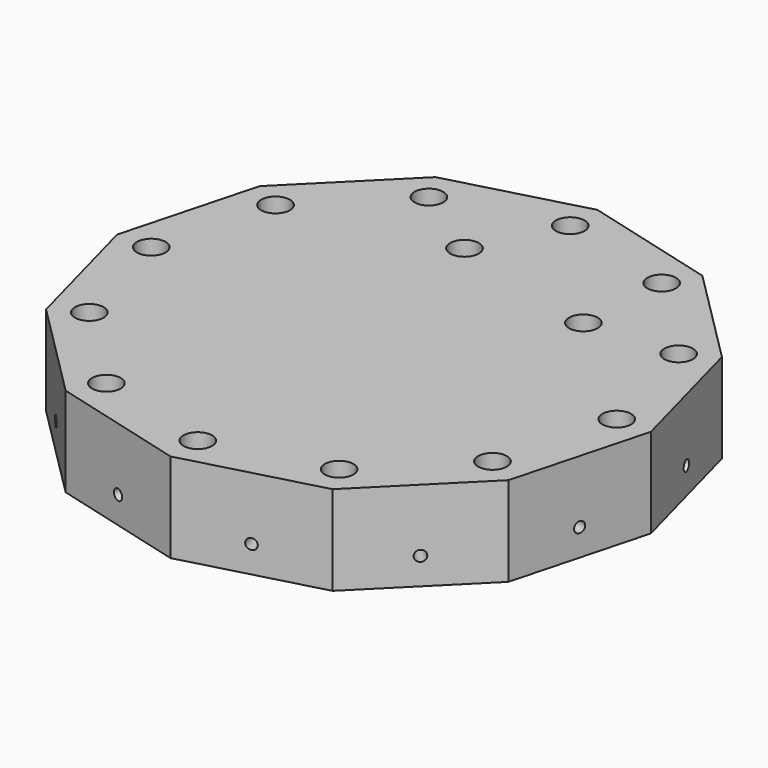
from build123d import *

# Parameters (mm, degrees)
F1_DEPTH  = 50
F2_R      = 8
F3_DEPTH  = 50
F4_COUNT  = 12
F4_ANGLE  = 330
F5_DEPTH  = 50.001
F6_DEPTH  = 25
F7_START  = 25
F7_DEPTH  = 25
F9_R      = 3
F10_DEPTH = 60
F11_DEPTH = 22
F12_COUNT = 9
F12_ANGLE = 240
F14_R     = 10
F15_DEPTH = 64
F16_R     = 10
F17_DEPTH = 64


# Not quite as in the source:
# - a feature names something its author has since deleted; it is built from what else it names


with BuildPart() as f1:
    # F0 (on Top) → F1 (new body)
    with BuildSketch(Plane.XY):
        Polygon((0, 149.0797699791), (-74.5398849895, 129.1068679922), (-129.1068679922, 74.5398849895), (-149.0797699791, 0), (-129.1068679922, -74.5398849895), (-74.5398849895, -129.1068679922), (0, -149.0797699791), (74.5398849895, -129.1068679922), (129.1068679922, -74.5398849895), (149.0797699791, 0), (129.1068679922, 74.5398849895), (74.5398849895, 129.1068679922), align=None)
    extrude(amount=F1_DEPTH)

    # F2 (on Top) → F5 (cut, through all)
    with BuildSketch(Plane.XY):
        with Locations((-22.6466664465, 84.5185098003)):
            Circle(F2_R)
    extrude(amount=F5_DEPTH, mode=Mode.SUBTRACT)

    # F2 (on Top) → F6 (cut)
    with BuildSketch(Plane.XY):
        with Locations((22.6466664465, 84.5185098003)):
            Circle(F2_R)
    extrude(amount=F6_DEPTH, mode=Mode.SUBTRACT)

    # F2 (on Top) → F7 (cut)
    with BuildSketch(Plane.XY.offset(F7_START)):
        with Locations((61.8718433538, 61.8718433538)):
            Circle(F2_R)
    extrude(amount=F7_DEPTH, mode=Mode.SUBTRACT)


with BuildPart() as f3:
    # F2 (on Top) → F3 (new body)
    with BuildSketch(Plane.XY):
        with Locations((0, 130)):
            Circle(F2_R)
    extrude(amount=F3_DEPTH)


with BuildPart() as f4_1:
    # F4: instance of F3
    add(f3.part.rotate(Axis((0, 0, 0), (0, 0, 1)), 1 * F4_ANGLE / (F4_COUNT - 1)))


with BuildPart() as f4_2:
    # F4: instance of F3
    add(f3.part.rotate(Axis((0, 0, 0), (0, 0, 1)), 2 * F4_ANGLE / (F4_COUNT - 1)))


with BuildPart() as f4_3:
    # F4: instance of F3
    add(f3.part.rotate(Axis((0, 0, 0), (0, 0, 1)), 3 * F4_ANGLE / (F4_COUNT - 1)))


with BuildPart() as f4_4:
    # F4: instance of F3
    add(f3.part.rotate(Axis((0, 0, 0), (0, 0, 1)), 4 * F4_ANGLE / (F4_COUNT - 1)))


with BuildPart() as f4_5:
    # F4: instance of F3
    add(f3.part.rotate(Axis((0, 0, 0), (0, 0, 1)), 5 * F4_ANGLE / (F4_COUNT - 1)))


with BuildPart() as f4_6:
    # F4: instance of F3
    add(f3.part.rotate(Axis((0, 0, 0), (0, 0, 1)), 6 * F4_ANGLE / (F4_COUNT - 1)))


with BuildPart() as f4_7:
    # F4: instance of F3
    add(f3.part.rotate(Axis((0, 0, 0), (0, 0, 1)), 7 * F4_ANGLE / (F4_COUNT - 1)))


with BuildPart() as f4_8:
    # F4: instance of F3
    add(f3.part.rotate(Axis((0, 0, 0), (0, 0, 1)), 8 * F4_ANGLE / (F4_COUNT - 1)))


with BuildPart() as f4_9:
    # F4: instance of F3
    add(f3.part.rotate(Axis((0, 0, 0), (0, 0, 1)), 9 * F4_ANGLE / (F4_COUNT - 1)))


with BuildPart() as f4_10:
    # F4: instance of F3
    add(f3.part.rotate(Axis((0, 0, 0), (0, 0, 1)), 10 * F4_ANGLE / (F4_COUNT - 1)))


with BuildPart() as f4_11:
    # F4: instance of F3
    add(f3.part.rotate(Axis((0, 0, 0), (0, 0, 1)), 11 * F4_ANGLE / (F4_COUNT - 1)))


with BuildPart() as f1_1:
    add(f1.part)

    # F8: cut F4_11, F4_10, F4_9, F4_8, F4_7, F4_6, F4_5, F4_4, F4_3, F4_2, F4_1, F3
    add(f4_11.part, mode=Mode.SUBTRACT)
    add(f4_10.part, mode=Mode.SUBTRACT)
    add(f4_9.part, mode=Mode.SUBTRACT)
    add(f4_8.part, mode=Mode.SUBTRACT)
    add(f4_7.part, mode=Mode.SUBTRACT)
    add(f4_6.part, mode=Mode.SUBTRACT)
    add(f4_5.part, mode=Mode.SUBTRACT)
    add(f4_4.part, mode=Mode.SUBTRACT)
    add(f4_3.part, mode=Mode.SUBTRACT)
    add(f4_2.part, mode=Mode.SUBTRACT)
    add(f4_1.part, mode=Mode.SUBTRACT)
    add(f3.part, mode=Mode.SUBTRACT)


with BuildPart() as f10:
    # F9 (on face) → F10 (new body, symmetric)
    with BuildSketch(Plane(origin=(-101.8233764909, 101.8233764909, 0), x_dir=(-0.7071067812, -0.7071067812, 0), z_dir=(-0.7071067812, 0.7071067812, 0))):
        with Locations((0, 15)):
            Circle(F9_R)
    extrude(amount=F10_DEPTH, both=True)


with BuildPart() as f11:
    # F2 (on Top) → F11 (new body, symmetric)
    with BuildSketch(Plane.XY):
        with Locations((-61.8718433538, 61.8718433538)):
            Circle(F2_R)
    extrude(amount=F11_DEPTH, both=True)


with BuildPart() as f12_1:
    # F12: instance of F10
    add(f10.part.rotate(Axis((0, 0, 0), (0, 0, 1)), 1 * F12_ANGLE / (F12_COUNT - 1)))


with BuildPart() as f12_2:
    # F12: instance of F10
    add(f10.part.rotate(Axis((0, 0, 0), (0, 0, 1)), 2 * F12_ANGLE / (F12_COUNT - 1)))


with BuildPart() as f12_3:
    # F12: instance of F10
    add(f10.part.rotate(Axis((0, 0, 0), (0, 0, 1)), 3 * F12_ANGLE / (F12_COUNT - 1)))


with BuildPart() as f12_4:
    # F12: instance of F10
    add(f10.part.rotate(Axis((0, 0, 0), (0, 0, 1)), 4 * F12_ANGLE / (F12_COUNT - 1)))


with BuildPart() as f12_5:
    # F12: instance of F10
    add(f10.part.rotate(Axis((0, 0, 0), (0, 0, 1)), 5 * F12_ANGLE / (F12_COUNT - 1)))


with BuildPart() as f12_6:
    # F12: instance of F10
    add(f10.part.rotate(Axis((0, 0, 0), (0, 0, 1)), 6 * F12_ANGLE / (F12_COUNT - 1)))


with BuildPart() as f12_7:
    # F12: instance of F10
    add(f10.part.rotate(Axis((0, 0, 0), (0, 0, 1)), 7 * F12_ANGLE / (F12_COUNT - 1)))


with BuildPart() as f12_8:
    # F12: instance of F10
    add(f10.part.rotate(Axis((0, 0, 0), (0, 0, 1)), 8 * F12_ANGLE / (F12_COUNT - 1)))


with BuildPart() as f12_9:
    # F12: instance of F11
    add(f11.part.rotate(Axis((0, 0, 0), (0, 0, 1)), 1 * F12_ANGLE / (F12_COUNT - 1)))


with BuildPart() as f12_10:
    # F12: instance of F11
    add(f11.part.rotate(Axis((0, 0, 0), (0, 0, 1)), 2 * F12_ANGLE / (F12_COUNT - 1)))


with BuildPart() as f12_11:
    # F12: instance of F11
    add(f11.part.rotate(Axis((0, 0, 0), (0, 0, 1)), 3 * F12_ANGLE / (F12_COUNT - 1)))


with BuildPart() as f12_12:
    # F12: instance of F11
    add(f11.part.rotate(Axis((0, 0, 0), (0, 0, 1)), 4 * F12_ANGLE / (F12_COUNT - 1)))


with BuildPart() as f12_13:
    # F12: instance of F11
    add(f11.part.rotate(Axis((0, 0, 0), (0, 0, 1)), 5 * F12_ANGLE / (F12_COUNT - 1)))


with BuildPart() as f12_14:
    # F12: instance of F11
    add(f11.part.rotate(Axis((0, 0, 0), (0, 0, 1)), 6 * F12_ANGLE / (F12_COUNT - 1)))


with BuildPart() as f12_15:
    # F12: instance of F11
    add(f11.part.rotate(Axis((0, 0, 0), (0, 0, 1)), 7 * F12_ANGLE / (F12_COUNT - 1)))


with BuildPart() as f12_16:
    # F12: instance of F11
    add(f11.part.rotate(Axis((0, 0, 0), (0, 0, 1)), 8 * F12_ANGLE / (F12_COUNT - 1)))


with BuildPart() as f1_2:
    add(f1_1.part)

    # F13: cut F10, F11, F12_1, F12_9, F12_2, F12_10, F12_3, F12_11, F12_4, F12_12, F12_5, F12_13, F12_14, F12_6, F12_15, F12_8, F12_16, F12_7
    add(f10.part, mode=Mode.SUBTRACT)
    add(f11.part, mode=Mode.SUBTRACT)
    add(f12_1.part, mode=Mode.SUBTRACT)
    add(f12_9.part, mode=Mode.SUBTRACT)
    add(f12_2.part, mode=Mode.SUBTRACT)
    add(f12_10.part, mode=Mode.SUBTRACT)
    add(f12_3.part, mode=Mode.SUBTRACT)
    add(f12_11.part, mode=Mode.SUBTRACT)
    add(f12_4.part, mode=Mode.SUBTRACT)
    add(f12_12.part, mode=Mode.SUBTRACT)
    add(f12_5.part, mode=Mode.SUBTRACT)
    add(f12_13.part, mode=Mode.SUBTRACT)
    add(f12_14.part, mode=Mode.SUBTRACT)
    add(f12_6.part, mode=Mode.SUBTRACT)
    add(f12_15.part, mode=Mode.SUBTRACT)
    add(f12_8.part, mode=Mode.SUBTRACT)
    add(f12_16.part, mode=Mode.SUBTRACT)
    add(f12_7.part, mode=Mode.SUBTRACT)

    # F14 (on face) → F15 (cut)
    with BuildSketch(Plane(origin=(101.8233764909, 101.8233764909, 0), x_dir=(-0.7071067812, 0.7071067812, 0), z_dir=(0.7071067812, 0.7071067812, 0))):
        with Locations((0, 25)):
            Circle(F14_R)
    extrude(amount=-F15_DEPTH, mode=Mode.SUBTRACT)

    # F16 (on face) → F17 (cut)
    with BuildSketch(Plane(origin=(37.2699424948, 139.0933189856, 0), x_dir=(-0.9659258263, 0.2588190451, 0), z_dir=(0.2588190451, 0.9659258263, 0))):
        with Locations((0, 25)):
            Circle(F16_R)
    extrude(amount=-F17_DEPTH, mode=Mode.SUBTRACT)


solid = f1_2.part
